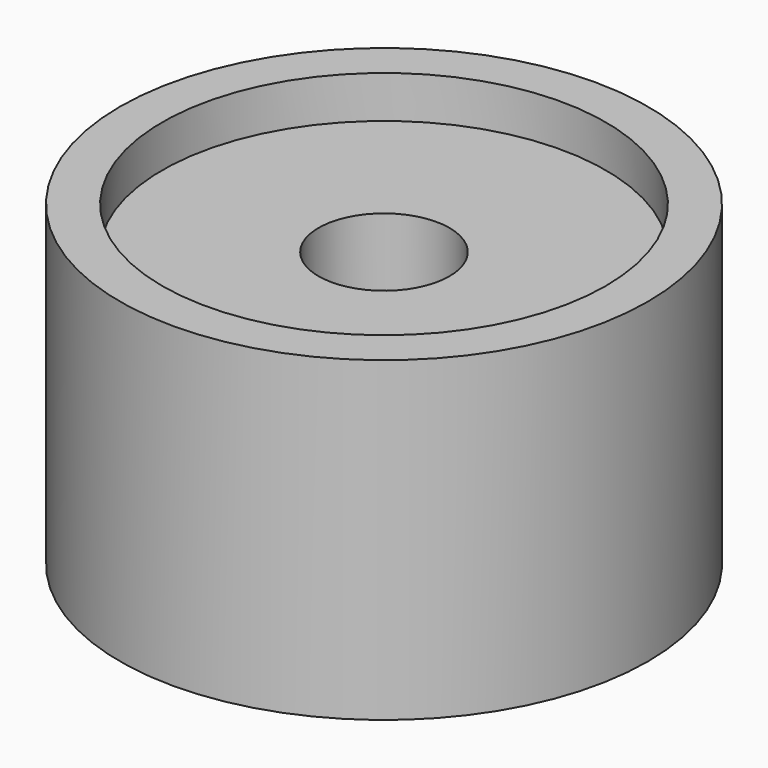
from build123d import *

# Parameters (mm, degrees)
F0_R     = 31.75
F1_DEPTH = 19.05
F2_R     = 26.67
F4_DEPTH = 5.08
F3_R     = 26.67
F5_DEPTH = 5.08
F6_R     = 7.874
F7_DEPTH = 50.8


with BuildPart() as f1:
    # F0 (on Top) → F1 (new body, symmetric)
    with BuildSketch(Plane.XY):
        Circle(F0_R)
    extrude(amount=F1_DEPTH, both=True)

    # F2 (on face) → F4 (cut)
    with BuildSketch(Plane.XY.offset(19.05)):
        Circle(F2_R)
    extrude(amount=-F4_DEPTH, mode=Mode.SUBTRACT)

    # F3 (on face) → F5 (cut)
    with BuildSketch(Plane(origin=(0, 0, -19.05), x_dir=(1, 0, 0), z_dir=(0, 0, -1))):
        Circle(F3_R)
    extrude(amount=-F5_DEPTH, mode=Mode.SUBTRACT)

    # F6 (on face) → F7 (cut)
    with BuildSketch(Plane.XY.offset(13.97)):
        Circle(F6_R)
    extrude(amount=-F7_DEPTH, mode=Mode.SUBTRACT)


solid = f1.part
